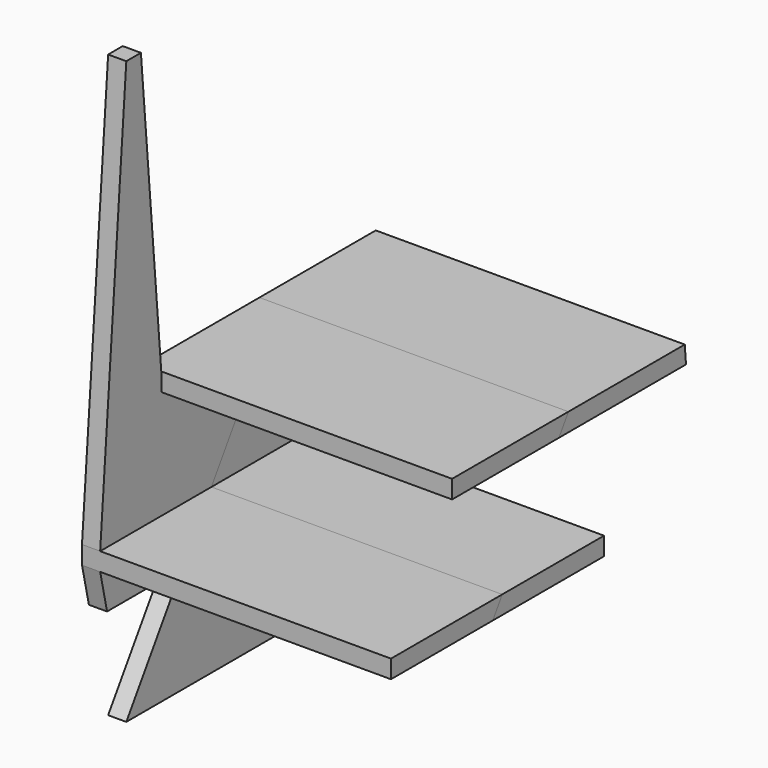
from build123d import *

# Parameters (mm, degrees)
F1_DEPTH = 25.4
F2_DEPTH = 25.4
F3_DEPTH = 406.4
F4_DEPTH = 406.4


with BuildPart() as f1:
    # F0 (on Right) → F1 (new body)
    with BuildSketch(Plane.YZ):
        Polygon((-637.9738673686, 228.6), (-538.8792110946, 381), (-725.5634350489, 381), (-748.838246869, 381), (-786.6158517795, 812.8), (-832.2896434142, 228.6), align=None)
        Polygon((-725.5634350489, 381), (-538.8792110946, 381), (-522.3634350489, 406.4), (-725.5634350489, 406.4), align=None)
        Polygon((-820.2121879405, 149.4681142857), (-689.4275879405, 149.4681142857), (-654.4896434142, 203.2), (-832.2896434142, 203.2), align=None)
        Polygon((-654.4896434142, 203.2), (-637.9738673686, 228.6), (-832.2896434142, 228.6), (-832.2896434142, 203.2), align=None)
        Polygon((-748.838246869, 381), (-725.5634350489, 381), (-725.5634350489, 406.4), (-761.1188279059, 812.8), (-786.6158517795, 812.8), align=None)
    extrude(amount=-F1_DEPTH)

    # F0 (on Right) → F3 (join)
    with BuildSketch(Plane.YZ):
        Polygon((-654.4896434142, 203.2), (-637.9738673686, 228.6), (-832.2896434142, 228.6), (-832.2896434142, 203.2), align=None)
        Polygon((-725.5634350489, 381), (-538.8792110946, 381), (-522.3634350489, 406.4), (-725.5634350489, 406.4), align=None)
    extrude(amount=F3_DEPTH)


with BuildPart() as f2:
    # F0 (on Right) → F2 (new body)
    with BuildSketch(Plane.YZ):
        Polygon((-319.1634350489, 0), (-283.608042192, 0), (-316.9412229954, 381), (-538.8792110946, 381), (-637.9738673686, 228.6), (-460.1738673686, 228.6), (-460.1738673686, 203.2), (-654.4896434142, 203.2), (-689.4275879405, 149.4681142857), (-786.6158517795, 0), align=None)
        Polygon((-538.8792110946, 381), (-316.9412229954, 381), (-319.1634350489, 406.4), (-522.3634350489, 406.4), align=None)
        Polygon((-460.1738673686, 228.6), (-637.9738673686, 228.6), (-654.4896434142, 203.2), (-460.1738673686, 203.2), align=None)
    extrude(amount=-F2_DEPTH)

    # F0 (on Right) → F4 (join)
    with BuildSketch(Plane.YZ):
        Polygon((-460.1738673686, 228.6), (-637.9738673686, 228.6), (-654.4896434142, 203.2), (-460.1738673686, 203.2), align=None)
        Polygon((-538.8792110946, 381), (-316.9412229954, 381), (-319.1634350489, 406.4), (-522.3634350489, 406.4), align=None)
    extrude(amount=F4_DEPTH)


solid = Compound([f1.part, f2.part])
